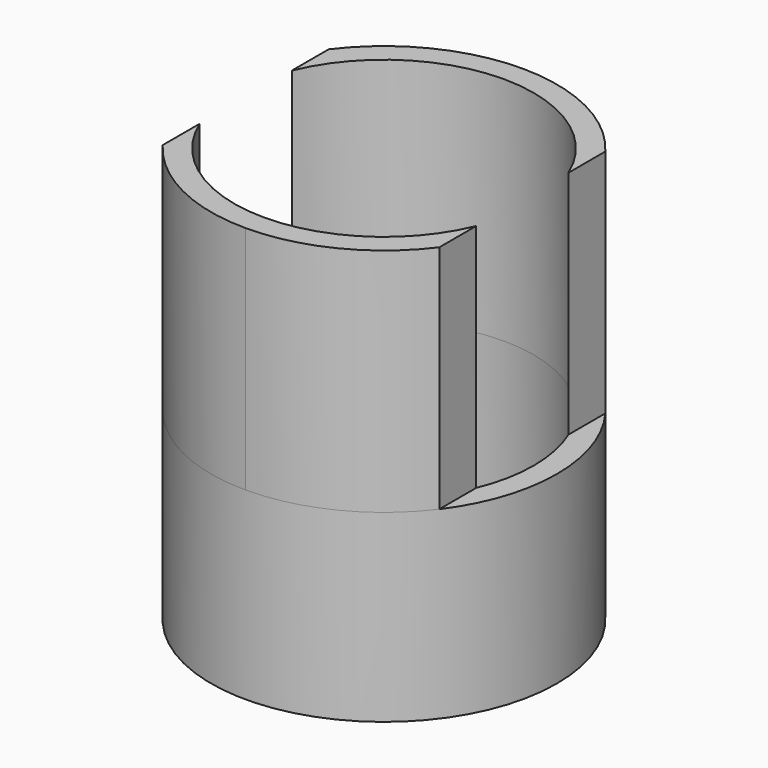
from build123d import *

# Parameters (mm, degrees)
F0_R     = 3.75
F1_DEPTH = 4
F3_DEPTH = 5
F4_DEPTH = 5


with BuildPart() as f1:
    # F0 (on Top) → F1 (new body)
    with BuildSketch(Plane.XY):
        Circle(F0_R)
    extrude(amount=F1_DEPTH)

    # F2 (on face) → F3 (cut, symmetric)
    with BuildSketch(Plane.XY.offset(4)):
        with BuildLine():
            ThreePointArc((3, -1.25), (3.186887196, -0.6373774392), (3.25, 0))
            ThreePointArc((3.25, 0), (3.186887196, 0.6373774392), (3, 1.25))
            ThreePointArc((3, 1.25), (0, 3.25), (-3, 1.25))
            ThreePointArc((-3, 1.25), (-3.25, 0), (-3, -1.25))
            ThreePointArc((-3, -1.25), (0, -3.25), (3, -1.25))
        make_face()
    extrude(amount=F3_DEPTH, both=True, mode=Mode.SUBTRACT)

    # F2 (on face) → F4 (join)
    with BuildSketch(Plane.XY.offset(4)):
        with BuildLine():
            ThreePointArc((-3, 1.25), (0, 3.25), (3, 1.25))
            Line((3, 1.25), (3, 2.25))
            ThreePointArc((3, 2.25), (1.6770509831, 3.3541019662), (0, 3.75))
            ThreePointArc((0, 3.75), (-1.6770509831, 3.3541019662), (-3, 2.25))
            Line((-3, 2.25), (-3, 1.25))
        make_face()
        with BuildLine():
            Line((3, -2.25), (3, -1.25))
            ThreePointArc((3, -1.25), (0, -3.25), (-3, -1.25))
            Line((-3, -1.25), (-3, -2.25))
            ThreePointArc((-3, -2.25), (-1.6770509831, -3.3541019662), (0, -3.75))
            ThreePointArc((0, -3.75), (1.6770509831, -3.3541019662), (3, -2.25))
        make_face()
    extrude(amount=F4_DEPTH)


solid = f1.part
